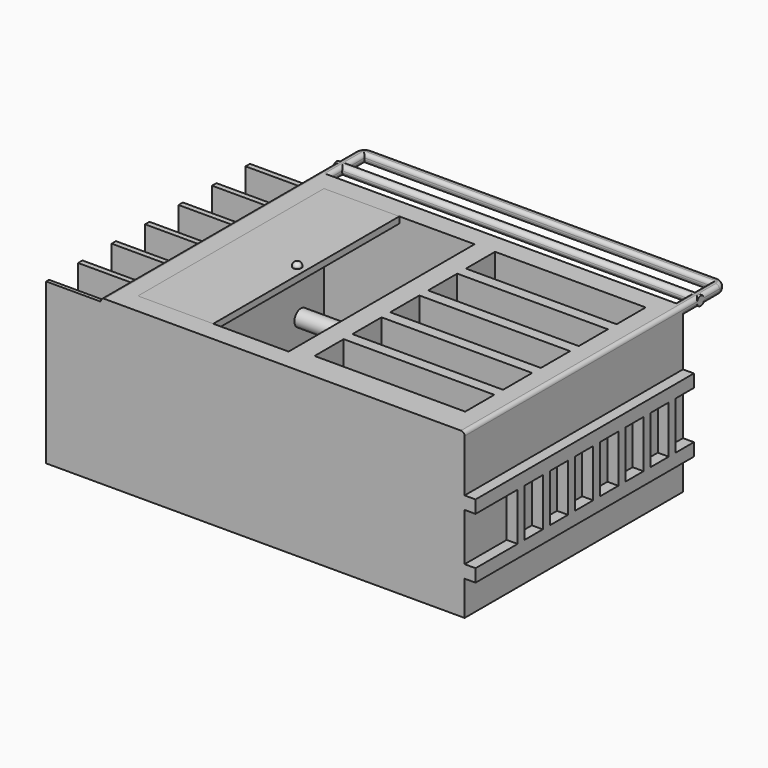
from build123d import *

# Parameters (mm, degrees)
F0_W      = 2000
F0_H      = 1500
F1_DEPTH  = 900
F2_W      = 1768.1858539581
F2_H      = 1277.7893543243
F3_DEPTH  = 740
F4_W      = 112.3773828149
F4_H      = 1277.7893543243
F5_DEPTH  = 740
F6_W      = 50
F6_H      = 50
F7_DEPTH  = 300
F9_W      = 50
F9_H      = 50
F10_DEPTH = 300
F8_W      = 50
F8_H      = 50
F11_DEPTH = 1933
F12_R     = 50
F13_R     = 50
F14_R     = 20
F16_DEPTH = 2000
F17_W     = 30
F17_H     = 880
F17_W_2   = 20
F18_DEPTH = 300
F19_R     = 45
F20_DEPTH = 929
F21_W     = 1836.2966775894
F21_H     = 732.2909879684
F22_DEPTH = 110
F23_W     = 827.9042355716
F23_H     = 50
F24_DEPTH = 550
F25_W     = 827.9042355716
F25_H     = 60
F25_H_2   = 37.7893543243
F26_DEPTH = 740
F27_W     = 1277.7893543243
F27_H     = 35
F28_DEPTH = 413.952
F29_R     = 22.5
F30_DEPTH = 25
F31_R     = 20
F32_W     = 48
F32_H     = 262.6869308949
F33_DEPTH = 60


with BuildPart() as f1:
    # F0 (on Top) → F1 (new body)
    with BuildSketch(Plane.XY):
        Rectangle(F0_W, F0_H)
    extrude(amount=F1_DEPTH)

    # F2 (on face) → F3 (cut)
    with BuildSketch(Plane.XY.offset(900)):
        Rectangle(F2_W, F2_H)
    extrude(amount=-F3_DEPTH, mode=Mode.SUBTRACT)

    # F4 (on face) → F5 (join)
    with BuildSketch(Plane.XY.offset(160)):
        Rectangle(F4_W, F4_H)
    extrude(amount=F5_DEPTH)

    # F6 (on face) → F7 (join)
    with BuildSketch(Plane(origin=(0, 750, 0), x_dir=(-1, 0, 0), z_dir=(0, 1, 0))):
        with Locations((-975, 875)):
            Rectangle(F6_W, F6_H)
    extrude(amount=F7_DEPTH)

    # F9 (on face) → F10 (join)
    with BuildSketch(Plane(origin=(0, 750, 0), x_dir=(-1, 0, 0), z_dir=(0, 1, 0))):
        with Locations((975, 875)):
            Rectangle(F9_W, F9_H)
    extrude(amount=F10_DEPTH)

    # F8 (on face) → F11 (join)
    with BuildSketch(Plane(origin=(950, 0, 0), x_dir=(0, -1, 0), z_dir=(-1, 0, 0))):
        with Locations((-1025, 875)):
            Rectangle(F8_W, F8_H)
    extrude(amount=F11_DEPTH)

    # F12
    f12_edges = [f1.edges().sort_by_distance(p)[0] for p in [
        (1000, 1050, 875),
    ]]
    fillet(f12_edges, radius=F12_R)

    # F13
    f13_edges = [f1.edges().sort_by_distance(p)[0] for p in [
        (-1000, 1050, 875),
    ]]
    fillet(f13_edges, radius=F13_R)

    # F14
    f14_edges = [f1.edges().sort_by_distance(p)[0] for p in [
        (-1000, 875, 850),
        (-950, 875, 900),
        (-950, 875, 850),
        (0, 1050, 900),
        (0, 1000, 900),
        (0, 1050, 850),
        (0, 1000, 850),
        (950, 875, 850),
        (950, 875, 900),
    ]]
    fillet(f14_edges, radius=F14_R)

    # F15 (on face) → F16 (join)
    with BuildSketch(Plane.YZ.offset(1000)):
        with BuildLine():
            Line((895.7658520367, 880), (871.2709546089, 880))
            Line((871.2709546089, 880), (871.2709546089, 870))
            Line((871.2709546089, 870), (895.7658520367, 870))
            ThreePointArc((895.7658520367, 870), (896.144358434, 872.4872759499), (896.2709546089, 875))
            ThreePointArc((896.2709546089, 875), (896.144358434, 877.5127240501), (895.7658520367, 880))
        make_face()
        with BuildLine():
            Line((846.7760571811, 880), (871.2709546089, 880))
            Line((871.2709546089, 880), (895.7658520367, 880))
            ThreePointArc((895.7658520367, 880), (871.2709546089, 900), (846.7760571811, 880))
        make_face()
        with BuildLine():
            Line((871.2709546089, 870), (871.2709546089, 880))
            Line((871.2709546089, 880), (846.7760571811, 880))
            ThreePointArc((846.7760571811, 880), (846.2709546089, 875), (846.7760571811, 870))
            Line((846.7760571811, 870), (871.2709546089, 870))
        make_face()
        with BuildLine():
            Line((895.7658520367, 870), (871.2709546089, 870))
            Line((871.2709546089, 870), (846.7760571811, 870))
            ThreePointArc((846.7760571811, 870), (871.2709546089, 850), (895.7658520367, 870))
        make_face()
    extrude(amount=-F16_DEPTH)

    # F17 (on face) → F18 (join)
    with BuildSketch(Plane(origin=(-1000, 0, 0), x_dir=(0, -1, 0), z_dir=(-1, 0, 0))):
        with Locations((-635, 440)):
            Rectangle(F17_W, F17_H)
        with Locations((-405, 440)):
            Rectangle(F17_W, F17_H)
        with Locations((-175, 440)):
            Rectangle(F17_W, F17_H)
        with Locations((55, 440)):
            Rectangle(F17_W, F17_H)
        with Locations((285, 440)):
            Rectangle(F17_W, F17_H)
        with Locations((515, 440)):
            Rectangle(F17_W, F17_H)
        with Locations((740, 440)):
            Rectangle(F17_W_2, F17_H)
    extrude(amount=F18_DEPTH)

    # F19 (on face) → F20 (join)
    with BuildSketch(Plane.YZ.offset(-884.0929269791)):
        with Locations((480.8457791805, 339.8399949074)):
            Circle(F19_R)
    extrude(amount=F20_DEPTH)

    # F21 (on face) → F22 (cut)
    with BuildSketch(Plane(origin=(0, 750, 0), x_dir=(-1, 0, 0), z_dir=(0, 1, 0))):
        with Locations((0, 435)):
            Rectangle(F21_W, F21_H)
    extrude(amount=-F22_DEPTH, mode=Mode.SUBTRACT)

    # F23 (on face) → F24 (join)
    with BuildSketch(Plane.XY.offset(160)):
        with Locations((-470.1408091933, -413.8946771622)):
            Rectangle(F23_W, F23_H)
    extrude(amount=F24_DEPTH)

    # F25 (on face) → F26 (join)
    with BuildSketch(Plane.XY.offset(160)):
        with Locations((470.1408091933, 408.8946771622)):
            Rectangle(F25_W, F25_H)
        with Locations((470.1408091933, 148.8946771622)):
            Rectangle(F25_W, F25_H)
        with Locations((470.1408091933, -111.1053228378)):
            Rectangle(F25_W, F25_H)
        with Locations((470.1408091933, -371.1053228378)):
            Rectangle(F25_W, F25_H)
        with Locations((470.1408091933, -620)):
            Rectangle(F25_W, F25_H_2)
    extrude(amount=F26_DEPTH)

    # F32 (on face) → F33 (join)
    with BuildSketch(Plane.YZ.offset(1000)):
        with Locations((601, 391.4981669188)):
            Rectangle(F32_W, F32_H)
        with Locations((428, 391.4981669188)):
            Rectangle(F32_W, F32_H)
        with Locations((255, 391.4981669188)):
            Rectangle(F32_W, F32_H)
        with Locations((82, 391.4981669188)):
            Rectangle(F32_W, F32_H)
        with Locations((-91, 391.4981669188)):
            Rectangle(F32_W, F32_H)
        with Locations((-264, 391.4981669188)):
            Rectangle(F32_W, F32_H)
        with Locations((-437, 391.4981669188)):
            Rectangle(F32_W, F32_H)
        Polygon((750, 190.1547014713), (750, 260.1547014713), (625, 260.1547014713), (577, 260.1547014713), (452, 260.1547014713), (404, 260.1547014713), (279, 260.1547014713), (231, 260.1547014713), (106, 260.1547014713), (58, 260.1547014713), (-67, 260.1547014713), (-115, 260.1547014713), (-240, 260.1547014713), (-288, 260.1547014713), (-413, 260.1547014713), (-461, 260.1547014713), (-750, 260.1547014713), (-750, 190.1547014713), align=None)
        Polygon((750, 522.8416323662), (750, 592.8416323662), (-750, 592.8416323662), (-750, 522.8416323662), (-461, 522.8416323662), (-413, 522.8416323662), (-288, 522.8416323662), (-240, 522.8416323662), (-115, 522.8416323662), (-67, 522.8416323662), (58, 522.8416323662), (106, 522.8416323662), (231, 522.8416323662), (279, 522.8416323662), (404, 522.8416323662), (452, 522.8416323662), (577, 522.8416323662), (625, 522.8416323662), align=None)
    extrude(amount=F33_DEPTH)


with BuildPart() as f28:
    # F27 (on face) → F28 (new body)
    with BuildSketch(Plane.YZ.offset(-884.0929269791)):
        with Locations((0, 882.5)):
            Rectangle(F27_W, F27_H)
    extrude(amount=F28_DEPTH)

    # F29 (on face) → F30 (join)
    with BuildSketch(Plane.XY.offset(900)):
        with Locations((-520.1409269791, 0)):
            Circle(F29_R)
    extrude(amount=F30_DEPTH)

    # F31
    f31_edges = [f28.edges().sort_by_distance(p)[0] for p in [
        (-542.640927, 0, 925),
    ]]
    fillet(f31_edges, radius=F31_R)


solid = Compound([f1.part, f28.part])
